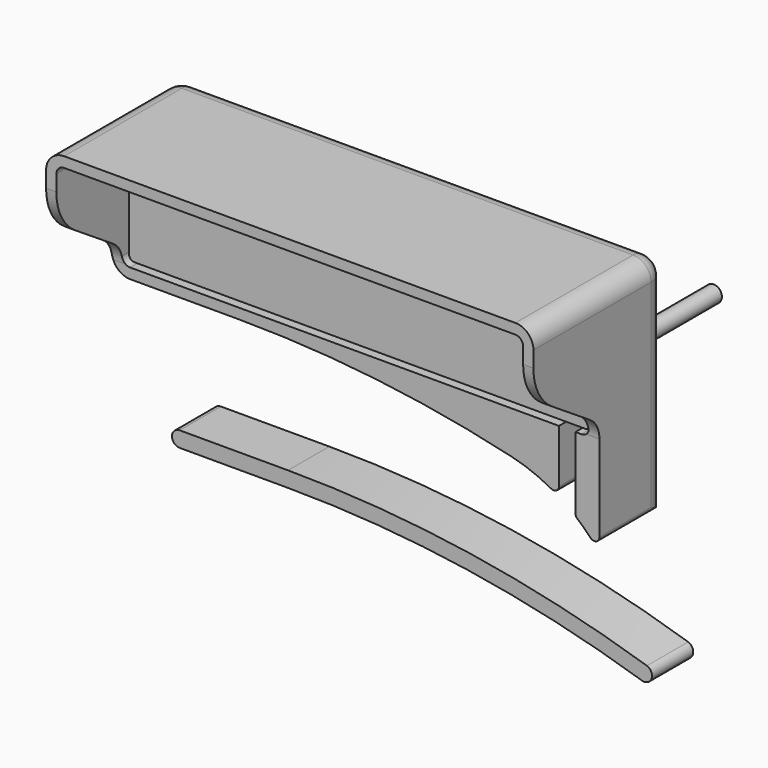
from build123d import *

# Parameters (mm, degrees)
F1_DEPTH      = 13
F3_DEPTH      = 3.5
F4_R          = 1.6
F5_DEPTH      = 25
F6_R          = 3.5
F7_DEPTH      = 2
F8_DEPTH      = 30
F10_DEPTH     = 94.501
F12_DEPTH     = 10
F13_T1_DEPTH  = 87.5
F13_T3_DEPTH  = 47.186229439
F13_T5_DEPTH  = 29.25
F13_T8_ANGLE  = 90
F13_T10_ANGLE = 90


# Not quite as in the source:
# - a fillet or chamfer that OpenCascade refuses, or shapes differently, is made with other operations: its cross-section is extruded or revolved along the edge and cut away or added


with BuildPart() as f1:
    # F0 (on Front) → F1 (new body)
    with BuildSketch(Plane.XZ):
        with BuildLine():
            Line((-43.75, -11.25), (43.75, -11.25))
            ThreePointArc((43.75, -11.25), (44.4571067812, -10.9571067812), (44.75, -10.25))
            Line((44.75, -10.25), (44.75, 10.25))
            ThreePointArc((44.75, 10.25), (44.4571067812, 10.9571067812), (43.75, 11.25))
            Line((43.75, 11.25), (-43.75, 11.25))
            ThreePointArc((-43.75, 11.25), (-44.4571067812, 10.9571067812), (-44.75, 10.25))
            Line((-44.75, 10.25), (-44.75, -10.25))
            ThreePointArc((-44.75, -10.25), (-44.4571067812, -10.9571067812), (-43.75, -11.25))
        make_face()
    extrude(amount=F1_DEPTH)

    # F2 (on face) → F3 (cut)
    with BuildSketch(Plane(origin=(0, 0, 0), x_dir=(-1, 0, 0), z_dir=(0, 1, 0))):
        with BuildLine():
            Line((-44.75, -1.35), (-44.75, -4.85))
            Line((-44.75, -4.85), (-41, -4.85))
            ThreePointArc((-41, -4.85), (-39.25, -3.1), (-41, -1.35))
            Line((-41, -1.35), (-44.75, -1.35))
        make_face()
    extrude(amount=-F3_DEPTH, mode=Mode.SUBTRACT)

    # F4 (on face) → F5 (join)
    with BuildSketch(Plane(origin=(0, -3.5, 0), x_dir=(-1, 0, 0), z_dir=(0, 1, 0))):
        with Locations((-41, -3.1)):
            Circle(F4_R)
    extrude(amount=F5_DEPTH)


with BuildPart() as f7:
    # F6 (on Front) → F7 (new body)
    with BuildSketch(Plane.XZ):
        with BuildLine():
            ThreePointArc((43.75, 11.75), (44.8106601718, 11.3106601718), (45.25, 10.25))
            Line((45.25, 10.25), (45.25, -1.35))
            Line((45.25, -1.35), (45.25, -4.85))
            Line((45.25, -4.85), (45.25, -10.25))
            ThreePointArc((45.25, -10.25), (44.8106601718, -11.3106601718), (43.75, -11.75))
            Line((43.75, -11.75), (42.6, -11.75))
            Line((42.6, -11.75), (42.6, -25.6736123026))
            ThreePointArc((42.6, -25.6736123026), (42.6929458463, -26.0946262718), (42.9545055245, -26.4373772417))
            ThreePointArc((42.9545055245, -26.4373772417), (44.2728453868, -27.6177334706), (45.5216463266, -28.8714308156))
            ThreePointArc((45.5216463266, -28.8714308156), (46.6185419424, -29.1158405602), (47.25, -28.186229439))
            Line((47.25, -28.186229439), (47.25, -23.3814297613))
            Line((47.25, -23.3814297613), (47.25, -10.25))
            Line((47.25, -10.25), (47.25, -4.85))
            Line((47.25, -4.85), (47.25, -1.35))
            Line((47.25, -1.35), (47.25, 10.25))
            ThreePointArc((47.25, 10.25), (46.2248737342, 12.7248737342), (43.75, 13.75))
            Line((43.75, 13.75), (-43.75, 13.75))
            ThreePointArc((-43.75, 13.75), (-46.2248737342, 12.7248737342), (-47.25, 10.25))
            Line((-47.25, 10.25), (-47.25, -10.25))
            ThreePointArc((-47.25, -10.25), (-46.2248737342, -12.7248737342), (-43.75, -13.75))
            Line((-43.75, -13.75), (-22.75, -13.75))
            ThreePointArc((-22.75, -13.75), (3.9329912025, -15.3151762113), (30.25, -19.9892369764))
            ThreePointArc((30.25, -19.9892369764), (34.1829257127, -21.2241281647), (37.917097158, -22.9702165145))
            ThreePointArc((37.917097158, -22.9702165145), (38.9084767241, -22.9556183115), (39.4, -22.0945425767))
            Line((39.4, -22.0945425767), (39.4, -11.75))
            Line((39.4, -11.75), (-43.75, -11.75))
            ThreePointArc((-43.75, -11.75), (-44.8106601718, -11.3106601718), (-45.25, -10.25))
            Line((-45.25, -10.25), (-45.25, 10.25))
            ThreePointArc((-45.25, 10.25), (-44.8106601718, 11.3106601718), (-43.75, 11.75))
            Line((-43.75, 11.75), (43.75, 11.75))
        make_face()
        with BuildLine():
            Line((45.25, -1.35), (45.25, 10.25))
            ThreePointArc((45.25, 10.25), (44.8106601718, 11.3106601718), (43.75, 11.75))
            Line((43.75, 11.75), (-43.75, 11.75))
            ThreePointArc((-43.75, 11.75), (-44.8106601718, 11.3106601718), (-45.25, 10.25))
            Line((-45.25, 10.25), (-45.25, -10.25))
            ThreePointArc((-45.25, -10.25), (-44.8106601718, -11.3106601718), (-43.75, -11.75))
            Line((-43.75, -11.75), (39.4, -11.75))
            Line((39.4, -11.75), (39.4, -4.4601470509))
            ThreePointArc((39.4, -4.4601470509), (41, -1), (42.6, -4.4601470509))
            Line((42.6, -4.4601470509), (42.6, -11.75))
            Line((42.6, -11.75), (43.75, -11.75))
            ThreePointArc((43.75, -11.75), (44.8106601718, -11.3106601718), (45.25, -10.25))
            Line((45.25, -10.25), (45.25, -4.85))
            Line((45.25, -4.85), (45.25, -1.35))
        make_face()
        with Locations((-31.75, 0)):
            Circle(F6_R, mode=Mode.SUBTRACT)
        with Locations((28, 0)):
            Circle(F6_R, mode=Mode.SUBTRACT)
    extrude(amount=-F7_DEPTH)

    # F6 (on Front) → F8 (join)
    with BuildSketch(Plane.XZ):
        with BuildLine():
            ThreePointArc((43.75, 11.75), (44.8106601718, 11.3106601718), (45.25, 10.25))
            Line((45.25, 10.25), (45.25, -1.35))
            Line((45.25, -1.35), (45.25, -4.85))
            Line((45.25, -4.85), (45.25, -10.25))
            ThreePointArc((45.25, -10.25), (44.8106601718, -11.3106601718), (43.75, -11.75))
            Line((43.75, -11.75), (42.6, -11.75))
            Line((42.6, -11.75), (42.6, -25.6736123026))
            ThreePointArc((42.6, -25.6736123026), (42.6929458463, -26.0946262718), (42.9545055245, -26.4373772417))
            ThreePointArc((42.9545055245, -26.4373772417), (44.2728453868, -27.6177334706), (45.5216463266, -28.8714308156))
            ThreePointArc((45.5216463266, -28.8714308156), (46.6185419424, -29.1158405602), (47.25, -28.186229439))
            Line((47.25, -28.186229439), (47.25, -23.3814297613))
            Line((47.25, -23.3814297613), (47.25, -10.25))
            Line((47.25, -10.25), (47.25, -4.85))
            Line((47.25, -4.85), (47.25, -1.35))
            Line((47.25, -1.35), (47.25, 10.25))
            ThreePointArc((47.25, 10.25), (46.2248737342, 12.7248737342), (43.75, 13.75))
            Line((43.75, 13.75), (-43.75, 13.75))
            ThreePointArc((-43.75, 13.75), (-46.2248737342, 12.7248737342), (-47.25, 10.25))
            Line((-47.25, 10.25), (-47.25, -10.25))
            ThreePointArc((-47.25, -10.25), (-46.2248737342, -12.7248737342), (-43.75, -13.75))
            Line((-43.75, -13.75), (-22.75, -13.75))
            ThreePointArc((-22.75, -13.75), (3.9329912025, -15.3151762113), (30.25, -19.9892369764))
            ThreePointArc((30.25, -19.9892369764), (34.1829257127, -21.2241281647), (37.917097158, -22.9702165145))
            ThreePointArc((37.917097158, -22.9702165145), (38.9084767241, -22.9556183115), (39.4, -22.0945425767))
            Line((39.4, -22.0945425767), (39.4, -11.75))
            Line((39.4, -11.75), (-43.75, -11.75))
            ThreePointArc((-43.75, -11.75), (-44.8106601718, -11.3106601718), (-45.25, -10.25))
            Line((-45.25, -10.25), (-45.25, 10.25))
            ThreePointArc((-45.25, 10.25), (-44.8106601718, 11.3106601718), (-43.75, 11.75))
            Line((-43.75, 11.75), (43.75, 11.75))
        make_face()
    extrude(amount=F8_DEPTH)

    # F9 (on face) → F10 (cut, through all)
    with BuildSketch(Plane.YZ.offset(47.25)):
        with BuildLine():
            Line((-30, -28.186229439), (-14, -28.186229439))
            Line((-14, -28.186229439), (-14, -11.4492685028))
            ThreePointArc((-14, -11.4492685028), (-14.6002039231, -9.074022309), (-16.2567177926, -7.2690289486))
            Line((-16.2567177926, -7.2690289486), (-25.4865644149, -1.2119421027))
            ThreePointArc((-25.4865644149, -1.2119421027), (-28.7995921539, 2.3980446179), (-30, 7.1485370056))
            Line((-30, 7.1485370056), (-30, -28.186229439))
        make_face()
        Polygon((-34.3077805638, -31.5740667284), (-14, -31.5740667284), (-14, -28.186229439), (-30, -28.186229439), (-30, 7.1485370056), (-30, 10.25), (-30, 16.696613282), (-34.3077805638, 16.696613282), align=None)
    extrude(amount=-F10_DEPTH, mode=Mode.SUBTRACT)

    # F13: fillet of radius 3.5 on 5 edges, made by hand

    # F13_s2 → F13_t1 (cut)
    with BuildSketch(Plane.YZ.offset(-43.75)):
        with BuildLine():
            ThreePointArc((2, 10.25), (0.9748737342, 12.7248737342), (-1.5, 13.75))
            Line((-1.5, 13.75), (2, 13.75))
            Line((2, 13.75), (2, 10.25))
        make_face()
    extrude(amount=F13_T1_DEPTH, mode=Mode.SUBTRACT)

    # F13_s4 → F13_t3 (cut)
    with BuildSketch(Plane.XY.offset(-36.936229439)):
        with BuildLine():
            ThreePointArc((43.75, 2), (46.2248737342, 0.9748737342), (47.25, -1.5))
            Line((47.25, -1.5), (47.25, 2))
            Line((47.25, 2), (43.75, 2))
        make_face()
    extrude(amount=F13_T3_DEPTH, mode=Mode.SUBTRACT)

    # F13_s6 → F13_t5 (cut)
    with BuildSketch(Plane.XY.offset(-19)):
        with BuildLine():
            ThreePointArc((-43.75, 2), (-46.2248737342, 0.9748737342), (-47.25, -1.5))
            Line((-47.25, -1.5), (-47.25, 2))
            Line((-47.25, 2), (-43.75, 2))
        make_face()
    extrude(amount=F13_T5_DEPTH, mode=Mode.SUBTRACT)

    # F13_s7 → F13_t8 (revolve, cut)
    with BuildSketch(Plane.XY.offset(10.25)):
        with BuildLine():
            ThreePointArc((43.75, 2), (46.2248737342, 0.9748737342), (47.25, -1.5))
            Line((47.25, -1.5), (47.25, 2))
            Line((47.25, 2), (43.75, 2))
        make_face()
    revolve(axis=Axis((43.75, 2, 10.25), (0, -1, 0)), revolution_arc=F13_T8_ANGLE, mode=Mode.SUBTRACT)

    # F13_s9 → F13_t10 (revolve, cut)
    with BuildSketch(Plane.YZ.offset(-43.75)):
        with BuildLine():
            ThreePointArc((2, 10.25), (0.9748737342, 12.7248737342), (-1.5, 13.75))
            Line((-1.5, 13.75), (2, 13.75))
            Line((2, 13.75), (2, 10.25))
        make_face()
    revolve(axis=Axis((-43.75, 2, 10.25), (0, -1, 0)), revolution_arc=F13_T10_ANGLE, mode=Mode.SUBTRACT)


with BuildPart() as f12:
    # F11 (on Front) → F12 (new body)
    with BuildSketch(Plane.XZ):
        with BuildLine():
            Line((-37.3423290549, -42.0881269919), (-16.3423290549, -42.0881269919))
            ThreePointArc((-16.3423290549, -42.0881269919), (18.412506359, -44.7499115968), (52.3566596423, -52.6731773254))
            ThreePointArc((52.3566596423, -52.6731773254), (54.169539989, -51.6724622056), (53.2596935507, -49.812315609))
            ThreePointArc((53.2596935507, -49.812315609), (18.8693514371, -41.7849002014), (-16.3423290549, -39.0881269919))
            Line((-16.3423290549, -39.0881269919), (-37.3423290549, -39.0881269919))
            ThreePointArc((-37.3423290549, -39.0881269919), (-38.8423290549, -40.5881269919), (-37.3423290549, -42.0881269919))
        make_face()
    extrude(amount=F12_DEPTH)


solid = Compound([f1.part, f7.part, f12.part])
